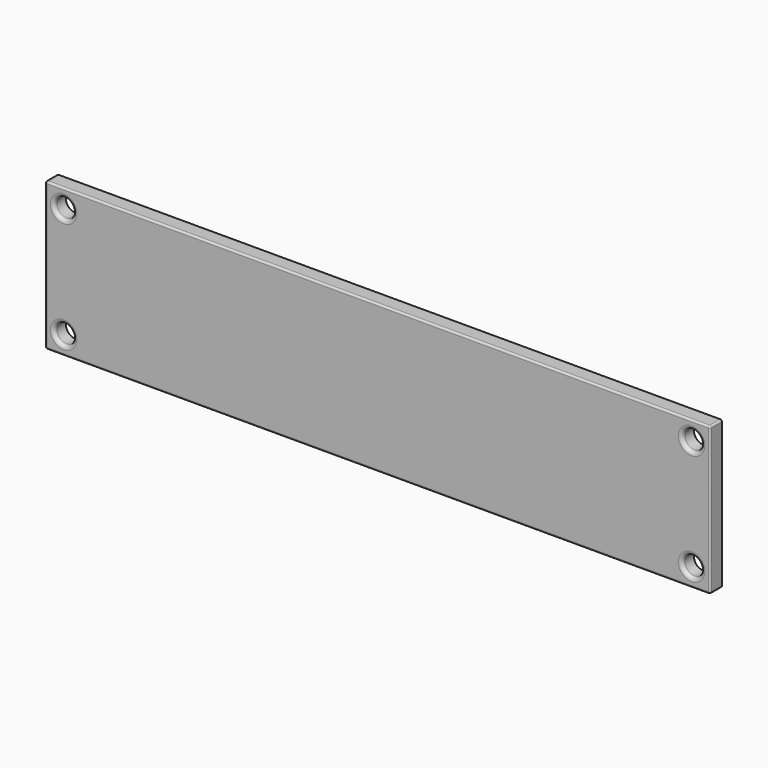
from build123d import *

# Parameters (mm, degrees)
F0_W         = 180
F0_H         = 40
F0_R         = 2.5751263091
F1_DEPTH     = 4
F2_R         = 1
F3_R         = 0.5
F4_TEXT_SIZE = 7.68
F5_DEPTH     = 1


# Not quite as in the source:
# - a feature names something its author has since deleted; it is built from what else it names
# - Text() gives the source's letters only with a copy of the font that has no kerning and outlines rounded to 1/6400 em; it was checked with that copy


with BuildPart() as f1:
    # F0 (on Front) → F1 (new body)
    with BuildSketch(Plane.XZ):
        Rectangle(F0_W, F0_H)
        with Locations((-85, -15)):
            Circle(F0_R, mode=Mode.SUBTRACT)
        with Locations((85, -15)):
            Circle(F0_R, mode=Mode.SUBTRACT)
        with Locations((-85, 15)):
            Circle(F0_R, mode=Mode.SUBTRACT)
        with Locations((85, 15)):
            Circle(F0_R, mode=Mode.SUBTRACT)
    extrude(amount=F1_DEPTH)

    # F2
    f2_edges = [f1.edges().sort_by_distance(p)[0] for p in [
        (-87.575126, -4, 15),
        (-87.575126, -4, -15),
        (82.424874, -4, 15),
        (82.424874, -4, -15),
    ]]
    fillet(f2_edges, radius=F2_R)

    # F3
    f3_edges = [f1.edges().sort_by_distance(p)[0] for p in [
        (0, -4, 20),
        (-90, -4, 0),
        (0, -4, -20),
        (90, -4, 0),
        (-90, -2, 20),
        (-90, -2, -20),
        (90, -2, 20),
        (90, -2, -20),
    ]]
    fillet(f3_edges, radius=F3_R)

    # F4 (on face) → F5 (join)
    with BuildSketch(Plane(origin=(0, 0, 0), x_dir=(-1, 0, 0), z_dir=(0, 1, 0))):
        with Locations((-70.5961091444, -2.7828512038)):
            Text('PS Cigar FP Body', F4_TEXT_SIZE, font='Open Sans', text_align=(TextAlign.LEFT, TextAlign.BOTTOM))
    extrude(amount=F5_DEPTH)

    # F6: F1 across plane


with BuildPart() as f1_1:
    add(f1.part)
    add(f1.part.mirror(Plane.YZ))


solid = f1_1.part
